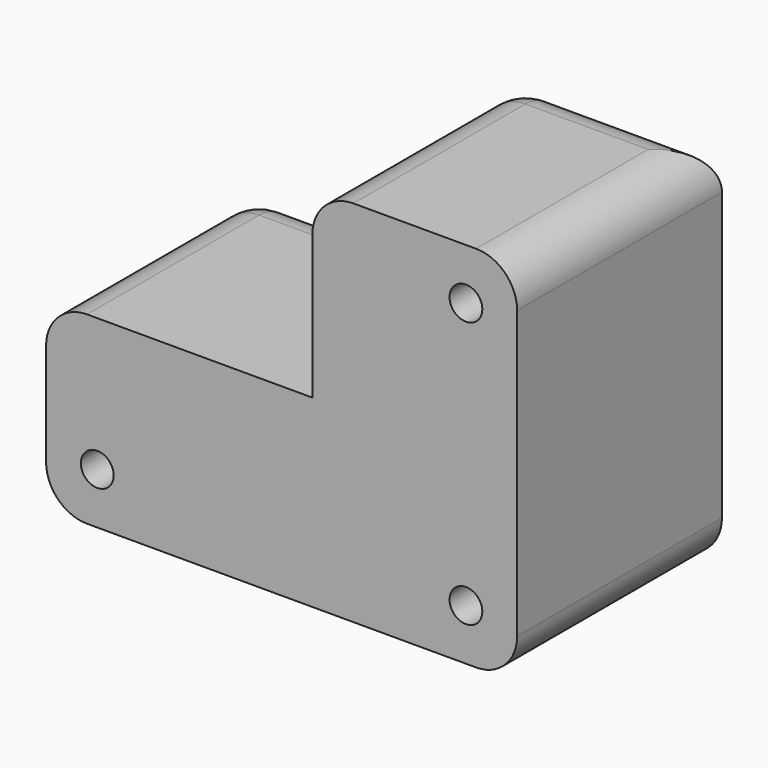
from build123d import *

# Parameters (mm, degrees)
F0_R         = 3.25
F0_R_2       = 1.6
F1_DEPTH     = 25
F2_DEPTH     = 15
F3_T1_DEPTH  = 24
F3_T3_DEPTH  = 22
F3_T5_DEPTH  = 14
F3_T7_DEPTH  = 26
F3_T9_DEPTH  = 31
F3_T11_DEPTH = 45
F3_S15_W     = 4
F3_S15_H     = 4
F3_T16_DEPTH = 4
F3_S21_W     = 4
F3_S21_H     = 4
F3_T22_DEPTH = 4
F3_T29_DEPTH = 32
F3_T33_DEPTH = 24


# Not quite as in the source:
# - a fillet or chamfer that OpenCascade refuses, or shapes differently, is made with other operations: its cross-section is extruded or revolved along the edge and cut away or added


with BuildPart() as f1:
    # F0 (on Front) → F1 (new body)
    with BuildSketch(Plane.XZ):
        Polygon((-23, 0), (-23, -18), (23, -18), (23, 18), (3, 18), (3, 0), align=None)
        with Locations((-18, -13)):
            Circle(F0_R, mode=Mode.SUBTRACT)
        with Locations((18, -13)):
            Circle(F0_R, mode=Mode.SUBTRACT)
        with Locations((18, 13)):
            Circle(F0_R, mode=Mode.SUBTRACT)
        with Locations((18, 13)):
            Circle(F0_R)
        with Locations((18, 13)):
            Circle(F0_R_2, mode=Mode.SUBTRACT)
        with Locations((18, -13)):
            Circle(F0_R)
        with Locations((18, -13)):
            Circle(F0_R_2, mode=Mode.SUBTRACT)
        with Locations((-18, -13)):
            Circle(F0_R)
        with Locations((-18, -13)):
            Circle(F0_R_2, mode=Mode.SUBTRACT)
    extrude(amount=F1_DEPTH)

    # F0 (on Front) → F2 (cut)
    with BuildSketch(Plane.XZ):
        with Locations((18, -13)):
            Circle(F0_R)
        with Locations((18, -13)):
            Circle(F0_R_2, mode=Mode.SUBTRACT)
        with Locations((-18, -13)):
            Circle(F0_R)
        with Locations((-18, -13)):
            Circle(F0_R_2, mode=Mode.SUBTRACT)
        with Locations((18, 13)):
            Circle(F0_R)
        with Locations((18, 13)):
            Circle(F0_R_2, mode=Mode.SUBTRACT)
    extrude(amount=F2_DEPTH, mode=Mode.SUBTRACT)

    # F3: fillet of radius 4 on 9 edges, made by hand

    # F3_s2 → F3_t1 (cut)
    with BuildSketch(Plane.XY.offset(-28)):
        with BuildLine():
            ThreePointArc((-23, -4), (-21.8284271247, -1.1715728753), (-19, 0))
            Line((-19, 0), (-23, 0))
            Line((-23, 0), (-23, -4))
        make_face()
    extrude(amount=F3_T1_DEPTH, mode=Mode.SUBTRACT)

    # F3_s4 → F3_t3 (cut)
    with BuildSketch(Plane.YZ.offset(-19)):
        with BuildLine():
            ThreePointArc((-4, 0), (-1.1715728753, -1.1715728753), (0, -4))
            Line((0, -4), (0, 0))
            Line((0, 0), (-4, 0))
        make_face()
    extrude(amount=F3_T3_DEPTH, mode=Mode.SUBTRACT)

    # F3_s6 → F3_t5 (cut)
    with BuildSketch(Plane.XY):
        with BuildLine():
            ThreePointArc((7, 0), (4.1715728753, -1.1715728753), (3, -4))
            Line((3, -4), (3, 0))
            Line((3, 0), (7, 0))
        make_face()
    extrude(amount=F3_T5_DEPTH, mode=Mode.SUBTRACT)

    # F3_s8 → F3_t7 (cut)
    with BuildSketch(Plane.YZ.offset(7)):
        with BuildLine():
            ThreePointArc((0, 14), (-1.1715728753, 16.8284271247), (-4, 18))
            Line((-4, 18), (0, 18))
            Line((0, 18), (0, 14))
        make_face()
    extrude(amount=F3_T7_DEPTH, mode=Mode.SUBTRACT)

    # F3_s10 → F3_t9 (cut)
    with BuildSketch(Plane.XZ.offset(4)):
        with BuildLine():
            ThreePointArc((-23, -4), (-21.8284271247, -1.1715728753), (-19, 0))
            Line((-19, 0), (-23, 0))
            Line((-23, 0), (-23, -4))
        make_face()
        with BuildLine():
            ThreePointArc((3, 14), (4.1715728753, 16.8284271247), (7, 18))
            Line((7, 18), (3, 18))
            Line((3, 18), (3, 14))
        make_face()
    extrude(amount=F3_T9_DEPTH, mode=Mode.SUBTRACT)

    # F3_s12 → F3_t11 (cut)
    with BuildSketch(Plane.XZ.offset(-10)):
        with BuildLine():
            ThreePointArc((-23, -14), (-21.8284271247, -16.8284271247), (-19, -18))
            Line((-19, -18), (-23, -18))
            Line((-23, -18), (-23, -14))
        make_face()
        with BuildLine():
            ThreePointArc((19, -18), (21.8284271247, -16.8284271247), (23, -14))
            Line((23, -14), (23, -18))
            Line((23, -18), (19, -18))
        make_face()
        with BuildLine():
            ThreePointArc((23, 14), (21.8284271247, 16.8284271247), (19, 18))
            Line((19, 18), (23, 18))
            Line((23, 18), (23, 14))
        make_face()
    extrude(amount=F3_T11_DEPTH, mode=Mode.SUBTRACT)


with BuildPart() as f3_tool14:
    # F3_s15 → F3_t16 (new body)
    with BuildSketch(Plane.YZ.offset(-19)):
        with Locations((-2, -2)):
            Rectangle(F3_S15_W, F3_S15_H)
    extrude(amount=-F3_T16_DEPTH)

    # F3_s17 → F3_t18 (revolve, cut)
    with BuildSketch(Plane(origin=(-19, -4, -4), x_dir=(0, -0.7071067812, -0.7071067812), z_dir=(0, 0.7071067812, -0.7071067812))):
        with BuildLine():
            ThreePointArc((0, -4), (4, 0), (0, 4))
            Line((0, 4), (0, -4))
        make_face()
    revolve(axis=Axis((-19, -4, -4), (-1, 0, 0)), mode=Mode.SUBTRACT)


with BuildPart() as f1_1:
    add(f1.part)

    # F3_t13: cut F3_tool14
    add(f3_tool14.part, mode=Mode.SUBTRACT)


with BuildPart() as f3_tool20:
    # F3_s21 → F3_t22 (new body)
    with BuildSketch(Plane.XZ.offset(4)):
        with Locations((5, 16)):
            Rectangle(F3_S21_W, F3_S21_H)
    extrude(amount=-F3_T22_DEPTH)

    # F3_s23 → F3_t24 (revolve, cut)
    with BuildSketch(Plane(origin=(7, -4, 14), x_dir=(0.7071067812, 0, -0.7071067812), z_dir=(0.7071067812, 0, 0.7071067812))):
        with BuildLine():
            ThreePointArc((0, -4), (4, 0), (0, 4))
            Line((0, 4), (0, -4))
        make_face()
    revolve(axis=Axis((7, -4, 14), (0, 1, 0)), mode=Mode.SUBTRACT)


with BuildPart() as f1_2:
    add(f1_1.part)

    # F3_t19: cut F3_tool20
    add(f3_tool20.part, mode=Mode.SUBTRACT)


with BuildPart() as f3_tool27:
    # F3_s28 → F3_t29 (new body)
    with BuildSketch(Plane.YZ.offset(13)):
        with BuildLine():
            ThreePointArc((-4, 0), (-1.1715728753, -1.1715728753), (0, -4))
            Line((0, -4), (0, 0))
            Line((0, 0), (-4, 0))
        make_face()
    extrude(amount=-F3_T29_DEPTH)

    split(bisect_by=Plane.YZ.offset(3), keep=Keep.TOP)


with BuildPart() as f3_tool31:
    # F3_s32 → F3_t33 (new body)
    with BuildSketch(Plane.XY.offset(14)):
        with BuildLine():
            ThreePointArc((7, 0), (4.1715728753, -1.1715728753), (3, -4))
            Line((3, -4), (3, 0))
            Line((3, 0), (7, 0))
        make_face()
    extrude(amount=-F3_T33_DEPTH)

    split(bisect_by=Plane.XY, keep=Keep.BOTTOM)


with BuildPart() as f3_tool27_1:
    add(f3_tool27.part)

    # F3_t35: intersect F3_tool31
    add(f3_tool31.part, mode=Mode.INTERSECT)


with BuildPart() as f1_3:
    add(f1_2.part)

    # F3_t25: cut F3_tool27
    add(f3_tool27_1.part, mode=Mode.SUBTRACT)


solid = f1_3.part
